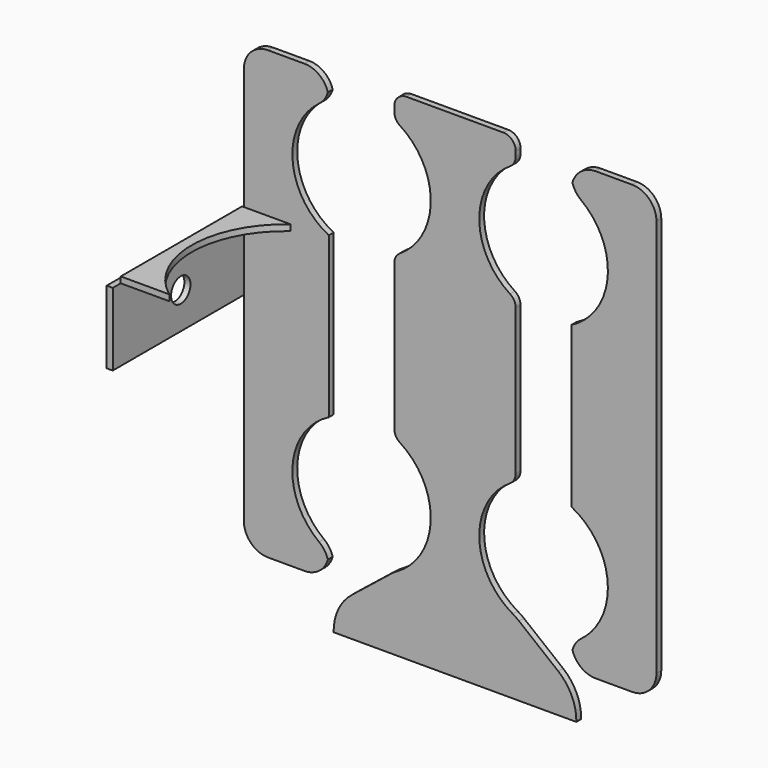
from build123d import *

# Parameters (mm, degrees)
F1_DEPTH      = 3.175
F2_T1_DEPTH   = 66.674967319
F2_T3_DEPTH   = 66.6750326811
F2_T5_DEPTH   = 38.1323821457
F2_T7_DEPTH   = 38.1378851793
F2_T9_DEPTH   = 66.675
F2_2_T1_DEPTH = 66.6749346379
F2_2_T3_DEPTH = 38.1476659019
F2_2_T5_DEPTH = 38.1421437691
F2_2_T7_DEPTH = 66.675
F2_2_T9_DEPTH = 66.6750326811
F4_DEPTH      = 3.175
F5_R          = 25.4
F6_R          = 6.35
F7_W          = 88.9
F7_H          = 38.1
F7_R          = 6.35
F8_DEPTH      = 3.175
F10_DEPTH     = 3.175


# Not quite as in the source:
# - a fillet or chamfer that OpenCascade refuses, or shapes differently, is made with other operations: its cross-section is extruded or revolved along the edge and cut away or added
# - ends of sketch curves that miss each other by under 0.0002 mm in the source are joined


with BuildPart() as f1:
    # F0 (on Front) → F1 (new body)
    with BuildSketch(Plane.XZ):
        with BuildLine():
            Line((-44.45, 25.4), (-44.4500065362, 12.7))
            Line((-44.4500065362, 12.7), (0, 12.7))
            Line((0, 12.7), (0, 246.3693658836))
            Line((0, 246.3693658836), (-44.4498862754, 246.3693658836))
            Line((-44.4498862754, 246.3693658836), (-44.4498928116, 233.6693658836))
            ThreePointArc((-44.4498928116, 233.6693658836), (-25.3953330127, 202.5585016842), (-44.4499248348, 171.4476570981))
            Line((-44.4499248348, 171.4476570981), (-44.4499679793, 87.6170231262))
            ThreePointArc((-44.4499679793, 87.6170231262), (-26.4276710435, 64.9184373675), (-31.7499999998, 36.4280565915))
            ThreePointArc((-31.7499999998, 36.4280565915), (-37.4261979997, 30.1380724116), (-44.45, 25.4))
        make_face()
    extrude(amount=F1_DEPTH)

    # F2: fillet of radius 12.7 on 6 edges, made by hand

    # F2_s2 → F2_t1 (cut)
    with BuildSketch(Plane.XZ.offset(-31.7499836595)):
        with BuildLine():
            ThreePointArc((-44.4498928116, 233.6693724198), (-40.7301466218, 242.6496243156), (-31.7498928116, 246.3693658836))
            Line((-31.7498928116, 246.3693658836), (-44.4498862754, 246.3693658836))
            Line((-44.4498862754, 246.3693658836), (-44.4498928116, 233.6693724198))
        make_face()
    extrude(amount=F2_T1_DEPTH, mode=Mode.SUBTRACT)

    # F2_s4 → F2_t3 (cut)
    with BuildSketch(Plane.XZ.offset(-31.7500163405)):
        with BuildLine():
            ThreePointArc((-44.45, 25.4000065362), (-40.730258432, 16.4197461898), (-31.75, 12.7))
            Line((-31.75, 12.7), (-44.4500065362, 12.7))
            Line((-44.4500065362, 12.7), (-44.45, 25.4000065362))
        make_face()
    extrude(amount=F2_T3_DEPTH, mode=Mode.SUBTRACT)

    # F2_s6 → F2_t5 (cut)
    with BuildSketch(Plane.XZ.offset(-17.4786910728)):
        with BuildLine():
            ThreePointArc((-44.4500035982, 18.4085235709), (-43.1092271942, 24.088133157), (-39.3700026387, 28.5685177543))
            ThreePointArc((-39.3700026387, 28.5685177543), (-41.8419793432, 26.8752011139), (-44.45, 25.4))
            Line((-44.45, 25.4), (-44.4500035982, 18.4085235709))
        make_face()
    extrude(amount=F2_T5_DEPTH, mode=Mode.SUBTRACT)

    # F2_s8 → F2_t7 (cut)
    with BuildSketch(Plane.XZ.offset(-17.4814425896)):
        with BuildLine():
            ThreePointArc((-39.3686742261, 230.5010252567), (-43.1087763961, 234.9816474858), (-44.4498892128, 240.6619429195))
            Line((-44.4498892128, 240.6619429195), (-44.4498928116, 233.6693658836))
            ThreePointArc((-44.4498928116, 233.6693658836), (-41.8412545983, 232.1942967863), (-39.3686742261, 230.5010252567))
        make_face()
    extrude(amount=F2_T7_DEPTH, mode=Mode.SUBTRACT)

    # F2_s10 → F2_t9 (cut)
    with BuildSketch(Plane.XZ.offset(-31.75)):
        with BuildLine():
            ThreePointArc((-12.7, 246.3693658836), (-3.7197438789, 242.6496220047), (0, 233.6693658836))
            Line((0, 233.6693658836), (0, 246.3693658836))
            Line((0, 246.3693658836), (-12.7, 246.3693658836))
        make_face()
        with BuildLine():
            ThreePointArc((0, 25.4), (-3.7197438789, 16.4197438789), (-12.7, 12.7))
            Line((-12.7, 12.7), (0, 12.7))
            Line((0, 12.7), (0, 25.4))
        make_face()
    extrude(amount=F2_T9_DEPTH, mode=Mode.SUBTRACT)


with BuildPart() as f1b:
    # F0 (on Front) → F1, piece 2 (new body)
    with BuildSketch(Plane.XZ):
        with BuildLine():
            Line((-171.4499549, 87.5937033957), (-171.4499117598, 171.4160283107))
            ThreePointArc((-171.4499117598, 171.4160283107), (-190.5080250242, 202.5287049682), (-171.4498797348, 233.6413620087))
            Line((-171.4498797348, 233.6413620087), (-171.4498731986, 246.3413620087))
            Line((-171.4498731986, 246.3413620087), (-215.8997464016, 246.3413848854))
            Line((-215.8997464016, 246.3413848854), (-215.8997464016, 12.6636870682))
            Line((-215.8997464016, 12.6636870682), (-171.4499999998, 12.6636870682))
            Line((-171.4499999998, 12.6636870682), (-171.4499869274, 25.3636870682))
            ThreePointArc((-171.4499869274, 25.3636870682), (-190.5126920115, 56.4787050428), (-171.4499549, 87.5937033957))
        make_face()
    extrude(amount=F1_DEPTH)

    # F2#2: fillet of radius 12.7 on 6 edges, made by hand

    # F2_2_s2 → F2_2_t1 (cut)
    with BuildSketch(Plane.XZ.offset(-31.749967319)):
        with BuildLine():
            ThreePointArc((-184.1499869274, 12.6636870682), (-175.1697354281, 16.3834263254), (-171.4499869274, 25.3636739958))
            Line((-171.4499869274, 25.3636739958), (-171.4499999998, 12.6636870682))
            Line((-171.4499999998, 12.6636870682), (-184.1499869274, 12.6636870682))
        make_face()
    extrude(amount=F2_2_T1_DEPTH, mode=Mode.SUBTRACT)

    # F2_2_s4 → F2_2_t3 (cut)
    with BuildSketch(Plane.XZ.offset(-17.486332951)):
        with BuildLine():
            ThreePointArc((-171.4499941271, 18.3691538878), (-172.7917123612, 24.050666351), (-176.5333802296, 28.5317056557))
            ThreePointArc((-176.5333802296, 28.5317056557), (-174.0597246836, 26.8385178049), (-171.4499869274, 25.3636870682))
            Line((-171.4499869274, 25.3636870682), (-171.4499941271, 18.3691538878))
        make_face()
    extrude(amount=F2_2_T3_DEPTH, mode=Mode.SUBTRACT)

    # F2_2_s6 → F2_2_t5 (cut)
    with BuildSketch(Plane.XZ.offset(-17.4835718845)):
        with BuildLine():
            ThreePointArc((-176.5320491725, 230.4731678841), (-172.7912596702, 234.9539670783), (-171.4498761355, 240.6347907625))
            Line((-171.4498761355, 240.6347907625), (-171.4498797348, 233.6413620087))
            ThreePointArc((-171.4498797348, 233.6413620087), (-174.058998545, 232.1663999192), (-176.5320491725, 230.4731678841))
        make_face()
    extrude(amount=F2_2_T5_DEPTH, mode=Mode.SUBTRACT)

    # F2_2_s8 → F2_2_t7 (cut)
    with BuildSketch(Plane.XZ.offset(-31.75)):
        with BuildLine():
            ThreePointArc((-171.4498797348, 233.6413620087), (-175.1696189919, 242.6216200442), (-184.1498731986, 246.3413685449))
            Line((-184.1498731986, 246.3413685449), (-171.4498731986, 246.3413620087))
            Line((-171.4498731986, 246.3413620087), (-171.4498797348, 233.6413620087))
        make_face()
        with BuildLine():
            ThreePointArc((-215.8997464016, 25.3636870682), (-212.1800025226, 16.3834309472), (-203.1997464016, 12.6636870682))
            Line((-203.1997464016, 12.6636870682), (-215.8997464016, 12.6636870682))
            Line((-215.8997464016, 12.6636870682), (-215.8997464016, 25.3636870682))
        make_face()
    extrude(amount=F2_2_T7_DEPTH, mode=Mode.SUBTRACT)

    # F2_2_s10 → F2_2_t9 (cut)
    with BuildSketch(Plane.XZ.offset(-31.7500163405)):
        with BuildLine():
            ThreePointArc((-203.1997398653, 246.3413783492), (-212.1800002117, 242.6216367812), (-215.8997464016, 233.6413783492))
            Line((-215.8997464016, 233.6413783492), (-215.8997464016, 246.3413848854))
            Line((-215.8997464016, 246.3413848854), (-203.1997398653, 246.3413783492))
        make_face()
    extrude(amount=F2_2_T9_DEPTH, mode=Mode.SUBTRACT)


with BuildPart() as f4:
    # F3 (on Front) → F4 (new body)
    with BuildSketch(Plane.XZ):
        with BuildLine():
            Line((-139.692944115, 171.4034480763), (-139.6929441151, 87.5811234915))
            ThreePointArc((-139.6929441151, 87.5811234915), (-120.6347981808, 56.4684481475), (-139.6929441152, 25.3557728035))
            Line((-139.6929441152, 25.3557728035), (-171.4463452584, -0.0442271965))
            Line((-171.4463452584, -0.0442271965), (-171.4463452584, -12.7442271965))
            Line((-171.4463452584, -12.7442271965), (-107.9463452584, -12.7442271965))
            Line((-107.9463452584, -12.7442271965), (-44.4463452584, -12.7442271965))
            Line((-44.4463452584, -12.7442271965), (-44.4463452584, -0.0442271965))
            Line((-44.4463452584, -0.0442271965), (-76.1997464016, 25.3897610103))
            ThreePointArc((-76.1997464016, 25.3897610103), (-95.2497464016, 56.4982807437), (-76.1997464016, 87.606800477))
            Line((-76.1997464016, 87.606800477), (-76.1997464016, 171.442142989))
            ThreePointArc((-76.1997464016, 171.442142989), (-95.2452147999, 202.548280738), (-76.1997464016, 233.6544184871))
            Line((-76.1997464016, 233.6544184871), (-76.1997464016, 246.3544184871))
            Line((-76.1997464016, 246.3544184871), (-139.692944115, 246.3544184871))
            Line((-139.692944115, 246.3544184871), (-139.692944115, 233.6334480764))
            ThreePointArc((-139.692944115, 233.6334480764), (-120.6302390309, 202.5184480763), (-139.692944115, 171.4034480763))
        make_face()
    extrude(amount=-F4_DEPTH)

    # F5
    f5_edges = [f4.edges().sort_by_distance(p)[0] for p in [
        (-171.446345, 1.5875, -0.044227),
        (-139.692944, 1.5875, 25.355773),
        (-76.199746, 1.5875, 25.389761),
        (-44.446345, 1.5875, -0.044227),
    ]]
    fillet(f5_edges, radius=F5_R)

    # F6
    f6_edges = [f4.edges().sort_by_distance(p)[0] for p in [
        (-139.692944, 1.5875, 246.354418),
        (-76.199746, 1.5875, 246.354418),
        (-76.199746, 1.5875, 233.654418),
        (-139.692944, 1.5875, 233.633448),
        (-139.692944, 1.5875, 171.403448),
        (-76.199746, 1.5875, 171.442143),
        (-76.199746, 1.5875, 87.6068),
        (-139.692944, 1.5875, 87.581123),
    ]]
    fillet(f6_edges, radius=F6_R)


with BuildPart() as f8:
    # F7 (on face) → F8 (new body)
    with BuildSketch(Plane(origin=(-215.8997464016, 0, 0), x_dir=(0, -1, 0), z_dir=(-1, 0, 0))):
        with Locations((44.45, 148.5525327087)):
            Rectangle(F7_W, F7_H)
        with Locations((44.45, 148.5525327087)):
            Circle(F7_R, mode=Mode.SUBTRACT)
    extrude(amount=F8_DEPTH)


with BuildPart() as f10:
    # F9 (on face) → F10 (new body)
    with BuildSketch(Plane.XY.offset(167.6025327087)):
        with BuildLine():
            Line((-190.4997464016, -4.3409317732), (-215.8997464016, -4.3409317732))
            Line((-215.8997464016, -4.3409317732), (-215.8997464016, -83.7159317732))
            Line((-215.8997464016, -83.7159317732), (-190.4997464016, -83.7159317732))
            ThreePointArc((-190.4997464016, -83.7159317732), (-210.5315857086, -44.0284317732), (-190.4997464016, -4.3409317732))
        make_face()
    extrude(amount=F10_DEPTH)


solid = Compound([f1.part, f1b.part, f4.part, f8.part, f10.part])
